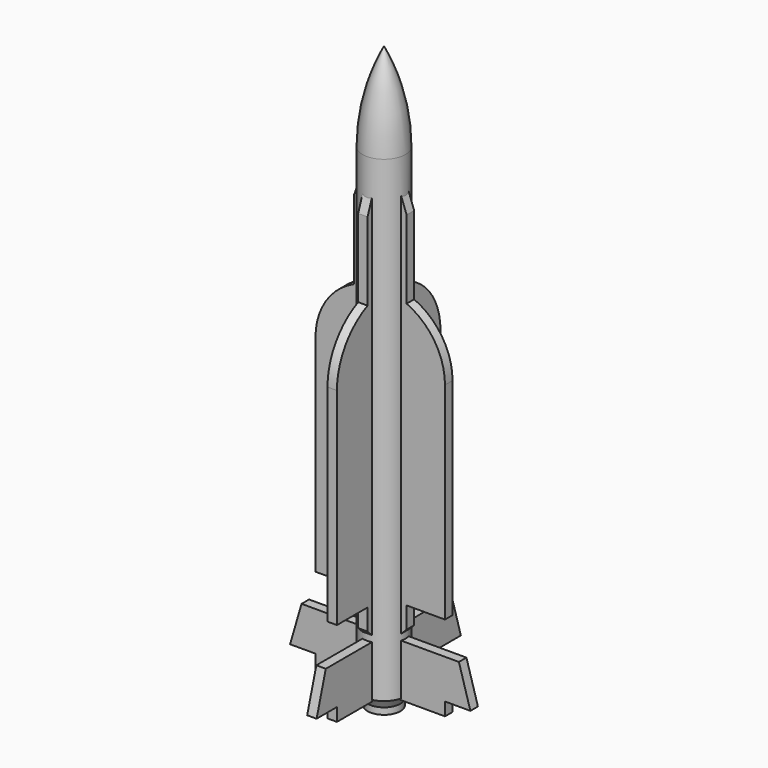
from build123d import *

# Parameters (mm, degrees)
F3_DEPTH = 0.2
F4_COUNT = 4


# Not quite as in the source:
# - a feature names something its author has since deleted; it is built from what else it names


with BuildPart() as f1:
    # F0 (on Front) → F1 (revolve)
    with BuildSketch(Plane.XZ):
        with BuildLine():
            Line((0, 24.5833333333), (0, 0))
            Line((0, 0), (0.6944444444, 0))
            Line((0.6944444444, 0), (0.6944444444, 0.2777777778))
            Line((0.6944444444, 0.2777777778), (0.9097222222, 0.625))
            Line((0.9097222222, 0.625), (0.9097222222, 20.8333333333))
            ThreePointArc((0.9097222222, 20.8333333333), (0.6790405117, 22.7627175953), (0, 24.5833333333))
        make_face()
    revolve(axis=Axis((0, 0, 12.2916666667), (0, 0, 1)))

    # F2 (on Front) → F3 (join, symmetric)
    with BuildSketch(Plane.XZ):
        with BuildLine():
            Line((0, 0.625), (0, 0.5555555556))
            Line((0, 0.5555555556), (2.7430555556, 0.5555555556))
            Line((2.7430555556, 0.5555555556), (2.7430555556, 1.1111111111))
            Line((2.7430555556, 1.1111111111), (3.8194444444, 1.1111111111))
            Line((3.8194444444, 1.1111111111), (3.3333333333, 2.7777777778))
            Line((3.3333333333, 2.7777777778), (0.8, 2.7777777778))
            Line((0.8, 2.7777777778), (0.8, 2.9458333333))
            Line((0.8, 2.9458333333), (1.1180555556, 3.2638888889))
            Line((1.1180555556, 3.2638888889), (1.1180555556, 4.1666666667))
            Line((1.1180555556, 4.1666666667), (2.7430555556, 4.1666666667))
            Line((2.7430555556, 4.1666666667), (2.7430555556, 12.9166666667))
            ThreePointArc((2.7430555556, 12.9166666667), (2.3012216629, 14.4095607148), (1.1180555556, 15.4215230609))
            Line((1.1180555556, 15.4215230609), (1.1180555556, 18.7331644265))
            Line((1.1180555556, 18.7331644265), (0, 21.8049968191))
            Line((0, 21.8049968191), (0, 0.625))
        make_face()
    extrude(amount=F3_DEPTH, both=True)

    # F4: F1 ×4 about axis
    f4_axis = Axis((0, 0, 0.625), (0, 0, 1))


with BuildPart() as f1_1:
    add(f1.part)
    for i in range(1, F4_COUNT):
        add(f1.part.rotate(f4_axis, i * 360 / F4_COUNT))


solid = f1_1.part
